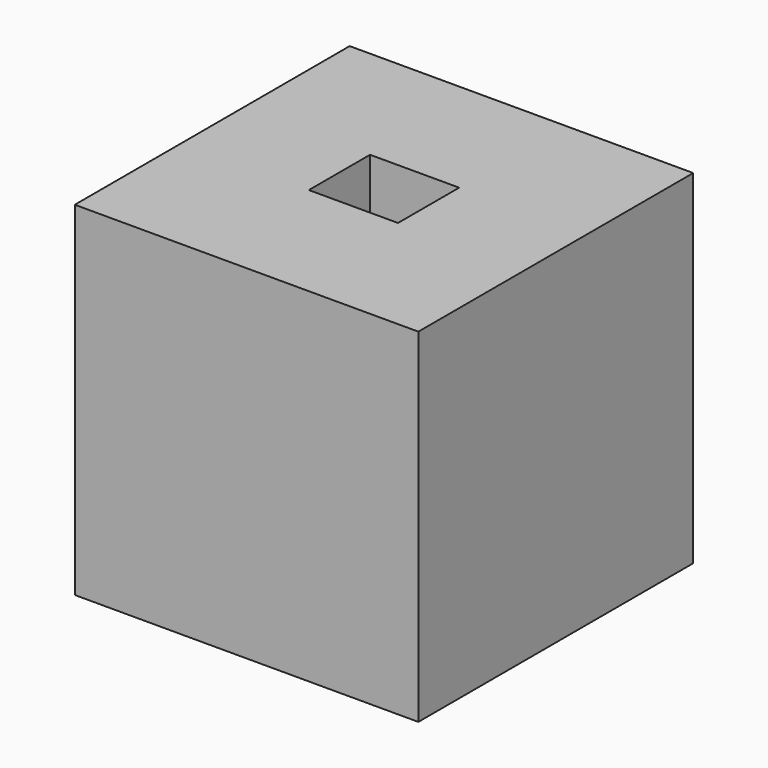
from build123d import *

# Parameters (mm, degrees)
F1_W     = 101.6
F1_H     = 101.6
F2_DEPTH = 50.8
F3_W     = 26.3578668237
F3_H     = 22.6122755557
F4_DEPTH = 50.8
F5_R     = 17.6293811016
F6_DEPTH = 50.8
F8_DEPTH = 50.8


# Not quite as in the source:
# - a variable given as a bare number and used for a length is read in inches; the dataset says mm whatever the document's units were


with BuildPart() as f2:
    # F1 (on Front) → F2 (new body, symmetric)
    with BuildSketch(Plane.XZ):
        Rectangle(F1_W, F1_H)
    extrude(amount=F2_DEPTH, both=True)

    # F3 (on face) → F4 (cut)
    with BuildSketch(Plane.XY.offset(50.8)):
        Rectangle(F3_W, F3_H)
    extrude(amount=-F4_DEPTH, mode=Mode.SUBTRACT)

    # F5 (on face) → F6 (cut)
    with BuildSketch(Plane(origin=(0, 0, -50.8), x_dir=(1, 0, 0), z_dir=(0, 0, -1))):
        with Locations((0, 1.7344856169)):
            Circle(F5_R)
    extrude(amount=-F6_DEPTH, mode=Mode.SUBTRACT)

    # F7 (on face) → F8 (cut)
    with BuildSketch(Plane(origin=(-50.8, 0, 0), x_dir=(0, -1, 0), z_dir=(-1, 0, 0))):
        Polygon((26.357864961, -15.2177204305), (26.357864961, 15.2177204305), (0, 30.435440861), (-26.357864961, 15.2177204305), (-26.357864961, -15.2177204305), (0, -30.435440861), align=None)
    extrude(amount=-F8_DEPTH, mode=Mode.SUBTRACT)


solid = f2.part
